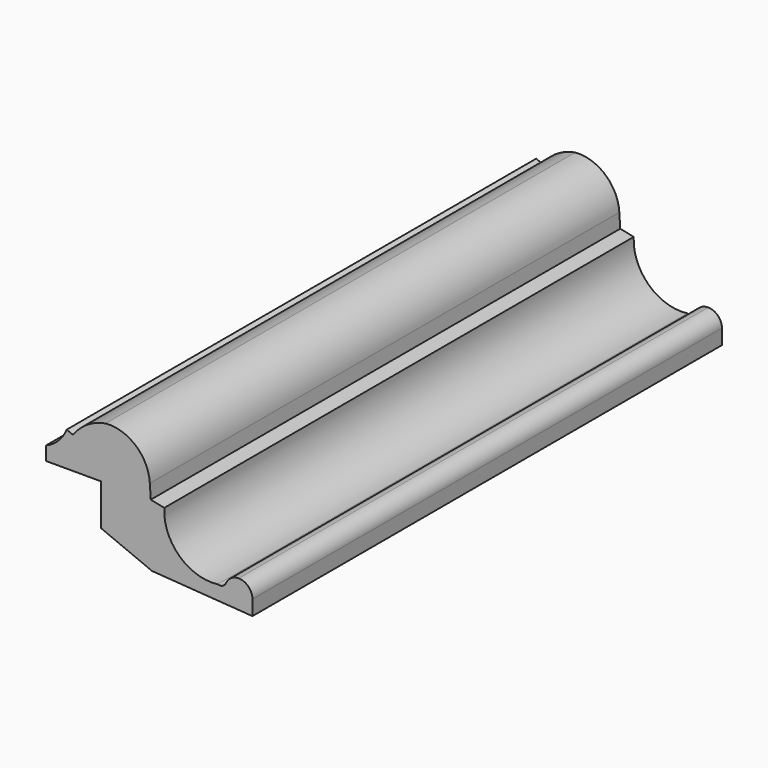
from build123d import *

# Parameters (mm, degrees)
F1_DEPTH = 152.4


# Not quite as in the source:
# - ends of sketch curves that miss each other by under 0.0002 mm in the source are joined


with BuildPart() as f1:
    # F0 (on Front) → F1 (new body)
    with BuildSketch(Plane.XZ):
        with BuildLine():
            ThreePointArc((-21.436008248, 11.1083378523), (-23.575890093, 7.8892124872), (-26.7950133579, 5.7493274827))
            Line((-26.7950133579, 5.7493274827), (-26.7950188, 2.1766784))
            Line((-26.7950188, 2.1766784), (-12.5043438, 2.1766784))
            Line((-12.5043438, 2.1766784), (-12.5043438, -8.5413342))
            Line((-12.5043438, -8.5413342), (0.6985, -14.010132))
            Line((0.6985, -14.010132), (26.7949934, -15.8565596))
            Line((26.7949934, -15.8565596), (26.7949934, -11.9503444))
            ThreePointArc((26.7949934, -11.9503444), (25.7485848099, -9.4240905901), (23.222331, -8.377682))
            ThreePointArc((23.222331, -8.377682), (21.2667719884, -8.9604103578), (19.949146016, -10.5185005939))
            ThreePointArc((19.949146016, -10.5185005939), (19.0509354729, -11.4291461184), (17.7741589903, -11.5058412669))
            ThreePointArc((17.7741589903, -11.5058412669), (7.8088470745, -8.265032818), (3.892042, 1.4544802))
            Line((3.892042, 1.4544802), (0.3963321215, 2.1892390214))
            Line((0.3963321215, 2.1892390214), (0.1486383408, 5.85559709))
            ThreePointArc((0.1486383408, 5.85559709), (-3.4794590188, 13.2572174827), (-11.3164912909, 15.8122126013))
            ThreePointArc((-11.3164912909, 15.8122126013), (-16.0919447869, 13.968734586), (-19.7856463188, 10.4247345468))
            Line((-19.7856463188, 10.4247345468), (-21.436008248, 11.1083378523))
        make_face()
    extrude(amount=F1_DEPTH)


solid = f1.part
